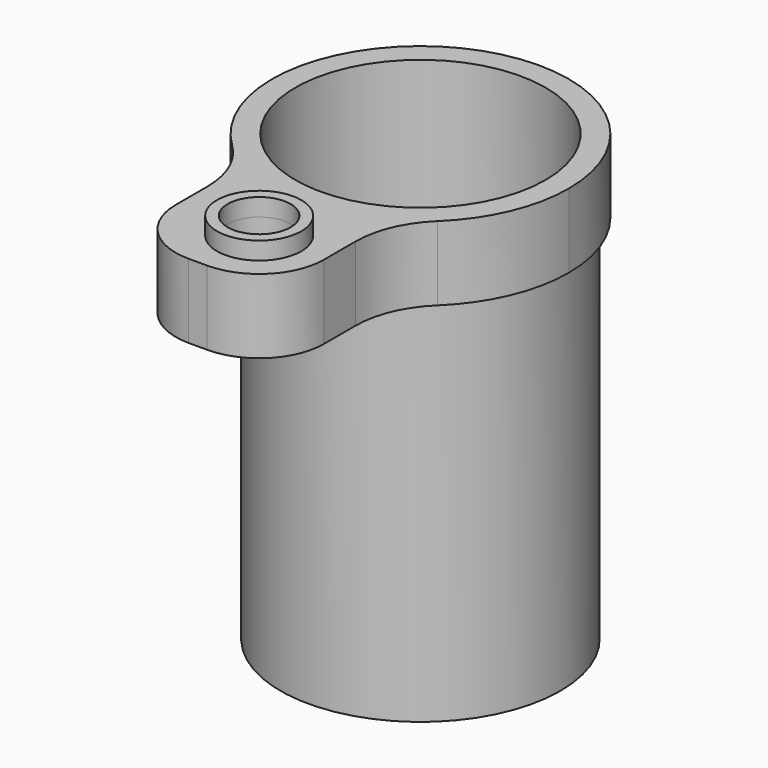
from build123d import *

# Parameters (mm, degrees)
F1_DEPTH  = 8
F2_R      = 15.1
F3_DEPTH  = 40
F4_R      = 7
F5_R      = 13.5
F6_DEPTH  = 46.5
F7_R      = 4.55
F7_R_2    = 3.4
F8_DEPTH  = 1.9
F9_DEPTH  = 48.001
F10_R     = 5.125
F10_R_2   = 3.4
F11_DEPTH = 3.75
F12_R     = 3
F13_DEPTH = 49.901
F14_R     = 10


with BuildPart() as f1:
    # F0 (on Top) → F1 (new body)
    with BuildSketch(Plane.XY):
        with BuildLine():
            ThreePointArc((8, -13.8564064606), (13.8564064606, -8), (16, 0))
            ThreePointArc((16, 0), (-8, 13.8564064606), (-8, -13.8564064606))
            Line((-8, -13.8564064606), (-8, 0))
            Line((-8, 0), (8, 0))
            Line((8, 0), (8, -13.8564064606))
        make_face()
        with BuildLine():
            Line((-8, 0), (-8, -13.8564064606))
            ThreePointArc((-8, -13.8564064606), (0, -16), (8, -13.8564064606))
            Line((8, -13.8564064606), (8, 0))
            Line((8, 0), (-8, 0))
        make_face()
        with BuildLine():
            ThreePointArc((8, -13.8564064606), (0, -16), (-8, -13.8564064606))
            Line((-8, -13.8564064606), (-8, -30))
            Line((-8, -30), (8, -30))
            Line((8, -30), (8, -13.8564064606))
        make_face()
    extrude(amount=F1_DEPTH)

    # F2 (on face) → F3 (join)
    with BuildSketch(Plane(origin=(0, 0, 0), x_dir=(1, 0, 0), z_dir=(0, 0, -1))):
        Circle(F2_R)
    extrude(amount=F3_DEPTH)

    # F4
    f4_edges = [f1.edges().sort_by_distance(p)[0] for p in [
        (-8, -30, 4),
        (8, -30, 4),
    ]]
    fillet(f4_edges, radius=F4_R)

    # F5 (on face) → F6 (cut)
    with BuildSketch(Plane.XY.offset(8)):
        Circle(F5_R)
    extrude(amount=-F6_DEPTH, mode=Mode.SUBTRACT)

    # F7 (on face) → F8 (join)
    with BuildSketch(Plane.XY.offset(8)):
        with Locations((1, -23)):
            Circle(F7_R)
        with Locations((1, -23)):
            Circle(F7_R_2, mode=Mode.SUBTRACT)
    extrude(amount=F8_DEPTH)

    # F9 (cut, through all): a face of the model
    f9_faces = [f1.faces().sort_by_distance(p)[0] for p in [
        (1, -23, 8),
    ]]
    extrude(f9_faces, amount=-F9_DEPTH, mode=Mode.SUBTRACT)

    # F10 (on face) → F11 (cut)
    with BuildSketch(Plane(origin=(0, 0, 0), x_dir=(1, 0, 0), z_dir=(0, 0, -1))):
        with Locations((1, 23)):
            Circle(F10_R)
        with Locations((1, 23)):
            Circle(F10_R_2, mode=Mode.SUBTRACT)
    extrude(amount=-F11_DEPTH, mode=Mode.SUBTRACT)

    # F12 (on face) → F13 (cut, through all)
    with BuildSketch(Plane(origin=(0, 0, -40), x_dir=(1, 0, 0), z_dir=(0, 0, -1))):
        Circle(F12_R)
    extrude(amount=-F13_DEPTH, mode=Mode.SUBTRACT)

    # F14
    f14_edges = [f1.edges().sort_by_distance(p)[0] for p in [
        (-8, -13.856406, 4),
        (8, -13.856406, 4),
    ]]
    fillet(f14_edges, radius=F14_R)


solid = f1.part
